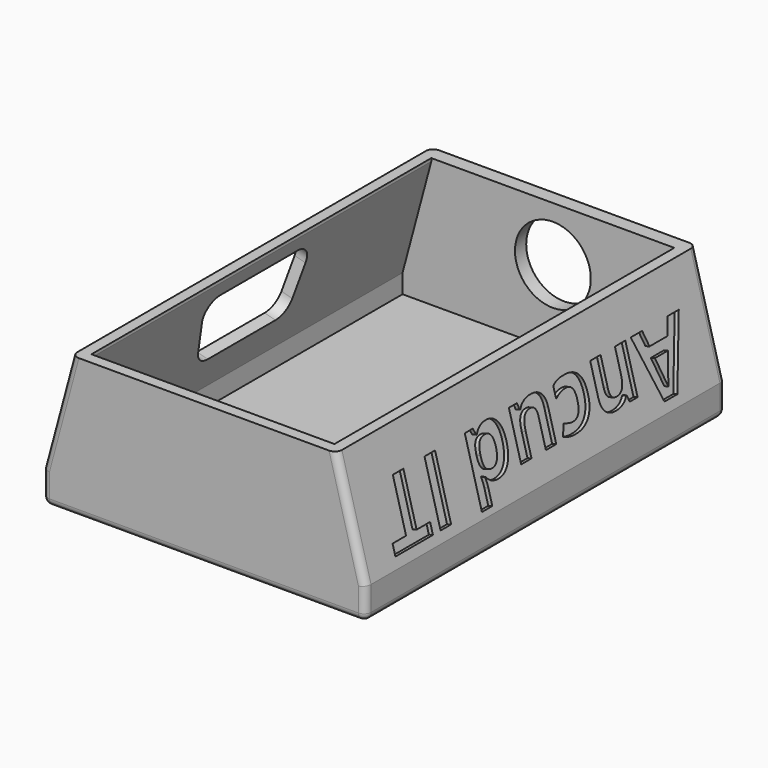
from build123d import *

# Parameters (mm, degrees)
F1_DEPTH      = 2
F3_DEPTH      = 60.5
F5_DEPTH      = 1.6
F6_R          = 5.4
F8_DEPTH      = 2
F9_R          = 1
F10_TEXT_SIZE = 12.3904952763
F11_DEPTH     = 0.6
F12_DEPTH     = 1.6000005166


# Not quite as in the source:
# - Text() gives the source's letters only with a copy of the font that has no kerning and outlines rounded to 1/6400 em; it was checked with that copy


with BuildPart() as f1:
    # F0 (on Front) → F1 (new body)
    with BuildSketch(Plane.XZ):
        Polygon((-23, 0), (23, 0), (23, 4.5), (18.8467875173, 20), (-18.8467875173, 20), (-23, 4.5), align=None)
    extrude(amount=F1_DEPTH)

    # F2 (on face) → F3 (join)
    with BuildSketch(Plane.XZ.offset(2)):
        Polygon((-23, 4.5), (-23, 0), (23, 0), (23, 4.5), (18.8467875173, 20), (17.3013056963, 20), (17.3013056963, 19.5858893941), (21.3999994834, 4.2893559359), (21.3999994834, 1.6000005166), (-21.3999994834, 1.6000005166), (-21.3999994834, 4.2893559359), (-17.3013056963, 19.5858893941), (-17.3013056963, 20), (-18.8467875173, 20), align=None)
    extrude(amount=F3_DEPTH)

    # F4 (on face) → F5 (join)
    with BuildSketch(Plane.XZ.offset(62.5)):
        Polygon((-23, 4.5), (-23, 0), (23, 0), (23, 4.5), (18.8467875173, 20), (-18.8467875173, 20), align=None)
    extrude(amount=F5_DEPTH)

    # F6 (on face) → F8 (cut, through all)
    with BuildSketch(Plane(origin=(0, 0, 0), x_dir=(-1, 0, 0), z_dir=(0, 1, 0))):
        with Locations((-0.0108149144, 12.25)):
            Circle(F6_R)
    extrude(amount=-F8_DEPTH, mode=Mode.SUBTRACT)

    # F9
    f9_edges = [f1.edges().sort_by_distance(p)[0] for p in [
        (20.923394, 0, 12.25),
        (-20.923394, 0, 12.25),
        (-20.923394, -64.1, 12.25),
        (20.923394, -64.1, 12.25),
        (0, -64.1, 0),
        (-23, -32.05, 0),
        (23, -32.05, 0),
        (0, 0, 0),
        (23, -64.1, 2.25),
        (-23, -64.1, 2.25),
        (23, 0, 2.25),
        (-23, 0, 2.25),
    ]]
    fillet(f9_edges, radius=F9_R)

    # F10 (on face) → F11 (cut)
    with BuildSketch(Plane(origin=(22.5842921435, 0, 6.0514428415), x_dir=(0, 1, 0), z_dir=(0.9659258263, 0, 0.2588190451))):
        with Locations(Location((-5, 8.6976212822), (0, 0, -180))):
            Text('Ancud IT', F10_TEXT_SIZE, font='Open Sans', font_style=FontStyle.BOLD, text_align=(TextAlign.LEFT, TextAlign.BOTTOM))
    extrude(amount=-F11_DEPTH, mode=Mode.SUBTRACT)

    # F7 (on face) → F12 (cut, through all)
    with BuildSketch(Plane(origin=(-22.5842921435, 0, 6.0514428415), x_dir=(0, -1, 0), z_dir=(-0.9659258263, 0, 0.2588190451))):
        with BuildLine():
            Line((38.8995386072, 12.4406089773), (25.1995386072, 12.4406089773))
            ThreePointArc((25.1995386072, 12.4406089773), (23.3610319437, 11.5832992405), (22.836, 9.6238533509))
            Line((22.836, 9.6238533509), (23.6647368093, 4.9238533509))
            ThreePointArc((23.6647368093, 4.9238533509), (24.4855851533, 3.5021023138), (26.0282754166, 2.9406089773))
            Line((26.0282754166, 2.9406089773), (38.0708017979, 2.9406089773))
            ThreePointArc((38.0708017979, 2.9406089773), (39.6134920611, 3.5021023138), (40.4343404051, 4.9238533509))
            Line((40.4343404051, 4.9238533509), (41.2630772145, 9.6238533509))
            ThreePointArc((41.2630772145, 9.6238533509), (40.7380452707, 11.5832992405), (38.8995386072, 12.4406089773))
        make_face()
    extrude(amount=-F12_DEPTH, mode=Mode.SUBTRACT)


solid = f1.part
